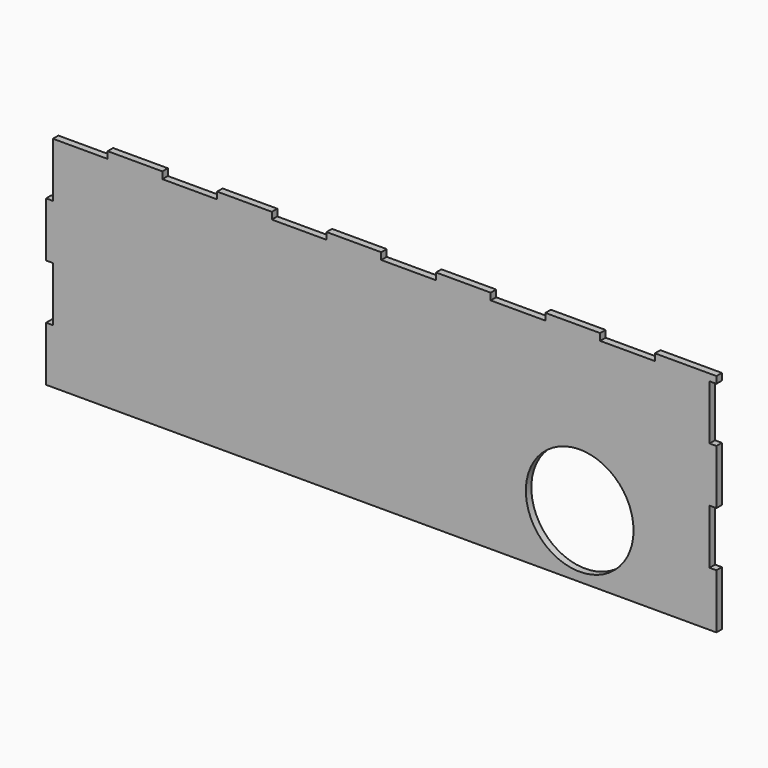
from build123d import *

# Parameters (mm, degrees)
F0_R     = 25
F1_DEPTH = 3.175


# Not quite as in the source:
# - a length typed as a fraction of an inch, garbled in the dataset ("3 / 203.2 mm" for 3/8 in), is restored


with BuildPart() as f1:
    # F0 (on Front) → F1 (new body)
    with BuildSketch(Plane.XZ):
        Polygon((-182.1372853069, 6.5356151886), (-178.9622853069, 6.5356151886), (125.8377146931, 6.5356151886), (129.0127146931, 6.5356151886), (129.0127146931, 31.9356151886), (125.8377146931, 31.9356151886), (125.8377146931, 57.3356151886), (129.0377632678, 57.3356151886), (129.0127146931, 82.7356151886), (125.8377146931, 82.7356151886), (125.8377146931, 108.1356151886), (129.0127146931, 108.1356151886), (129.0127146931, 111.3106151886), (125.8377146931, 111.3106151886), (100.4377146931, 111.3106151886), (100.4377146931, 108.1356151886), (75.0377146931, 108.1356151886), (75.0377146931, 111.3106151886), (49.6377146931, 111.3106151886), (49.6377146931, 108.1356151886), (24.2377146931, 108.1356151886), (24.2377146931, 111.3106151886), (-1.1622853069, 111.3106151886), (-1.1622853069, 108.1356151886), (-26.5622853069, 108.1356151886), (-26.5622853069, 111.3106151886), (-51.9622853069, 111.3106151886), (-51.9622853069, 108.1356151886), (-77.3622853069, 108.1356151886), (-77.3622853069, 111.3106151886), (-102.7622853069, 111.3106151886), (-102.7622853069, 108.1356151886), (-128.1622853069, 108.1356151886), (-128.1622853069, 111.3106151886), (-153.5622853069, 111.3106151886), (-153.5622853069, 108.1356151886), (-178.9622853069, 108.1356151886), (-178.9622853069, 82.7356151886), (-182.1372853069, 82.7356151886), (-182.1372853069, 57.3356151886), (-178.9622853069, 57.3356151886), (-178.9622853069, 31.9356151886), (-182.1372853069, 31.9356151886), align=None)
        with Locations((65.5590817332, 35.6867462397)):
            Circle(F0_R, mode=Mode.SUBTRACT)
    extrude(amount=F1_DEPTH)


solid = f1.part
